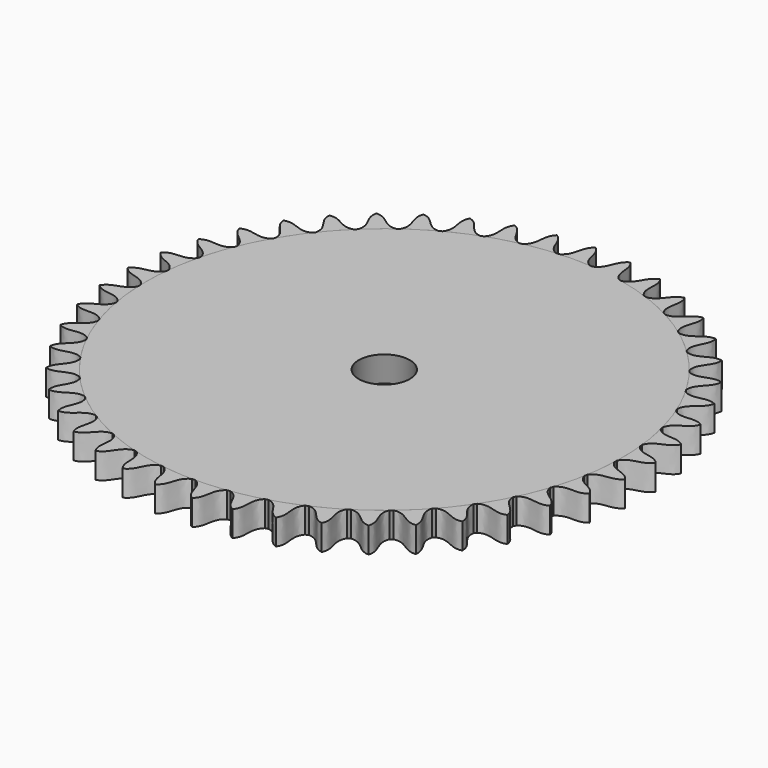
from build123d import *

# Parameters (mm, degrees)
F2_R     = 6
F2_R_2   = 4
F3_DEPTH = 4
F4_COUNT = 45


with BuildPart() as f3:
    # F2 (on Top) → F3 (new body)
    with BuildSketch(Plane.XY):
        with BuildLine():
            ThreePointArc((-2.3528037666, 37.167862426), (-25.4888403137, -27.1533552686), (37.2422566835, 0))
            ThreePointArc((37.2422566835, 0), (27.1533552686, 25.4888403137), (2.3528037666, 37.167862426))
            ThreePointArc((2.3528037666, 37.167862426), (0, 37.2422566835), (-2.3528037666, 37.167862426))
        make_face()
        Circle(F2_R, mode=Mode.SUBTRACT)
        Circle(F2_R)
        Circle(F2_R_2, mode=Mode.SUBTRACT)
        with BuildLine():
            ThreePointArc((-2.3528037666, 37.167862426), (0, 37.2422566835), (2.3528037666, 37.167862426))
            add(Edge.make_bspline(
                [(0, 41.294973545), (1.5, 40.167862426), (0.65, 38.167862426), (2.3528037666, 37.167862426)],
                knots=[0, 0, 0, 0, 4.7506559287, 4.7506559287, 4.7506559287, 4.7506559287], degree=3))
            add(Edge.make_bspline(
                [(0, 41.294973545), (-1.5, 40.167862426), (-0.65, 38.167862426), (-2.3528037666, 37.167862426)],
                knots=[0, 0, 0, 0, 4.7506559287, 4.7506559287, 4.7506559287, 4.7506559287], degree=3))
        make_face()
    extrude(amount=F3_DEPTH)


with BuildPart() as f4_1:
    # F4: instance of F3
    add(f3.part.rotate(Axis((0, 0, 4), (0, 0, 1)), 1 * 360 / F4_COUNT))


with BuildPart() as f4_2:
    # F4: instance of F3
    add(f3.part.rotate(Axis((0, 0, 4), (0, 0, 1)), 2 * 360 / F4_COUNT))


with BuildPart() as f4_3:
    # F4: instance of F3
    add(f3.part.rotate(Axis((0, 0, 4), (0, 0, 1)), 3 * 360 / F4_COUNT))


with BuildPart() as f4_4:
    # F4: instance of F3
    add(f3.part.rotate(Axis((0, 0, 4), (0, 0, 1)), 4 * 360 / F4_COUNT))


with BuildPart() as f4_5:
    # F4: instance of F3
    add(f3.part.rotate(Axis((0, 0, 4), (0, 0, 1)), 5 * 360 / F4_COUNT))


with BuildPart() as f4_6:
    # F4: instance of F3
    add(f3.part.rotate(Axis((0, 0, 4), (0, 0, 1)), 6 * 360 / F4_COUNT))


with BuildPart() as f4_7:
    # F4: instance of F3
    add(f3.part.rotate(Axis((0, 0, 4), (0, 0, 1)), 7 * 360 / F4_COUNT))


with BuildPart() as f4_8:
    # F4: instance of F3
    add(f3.part.rotate(Axis((0, 0, 4), (0, 0, 1)), 8 * 360 / F4_COUNT))


with BuildPart() as f4_9:
    # F4: instance of F3
    add(f3.part.rotate(Axis((0, 0, 4), (0, 0, 1)), 9 * 360 / F4_COUNT))


with BuildPart() as f4_10:
    # F4: instance of F3
    add(f3.part.rotate(Axis((0, 0, 4), (0, 0, 1)), 10 * 360 / F4_COUNT))


with BuildPart() as f4_11:
    # F4: instance of F3
    add(f3.part.rotate(Axis((0, 0, 4), (0, 0, 1)), 11 * 360 / F4_COUNT))


with BuildPart() as f4_12:
    # F4: instance of F3
    add(f3.part.rotate(Axis((0, 0, 4), (0, 0, 1)), 12 * 360 / F4_COUNT))


with BuildPart() as f4_13:
    # F4: instance of F3
    add(f3.part.rotate(Axis((0, 0, 4), (0, 0, 1)), 13 * 360 / F4_COUNT))


with BuildPart() as f4_14:
    # F4: instance of F3
    add(f3.part.rotate(Axis((0, 0, 4), (0, 0, 1)), 14 * 360 / F4_COUNT))


with BuildPart() as f4_15:
    # F4: instance of F3
    add(f3.part.rotate(Axis((0, 0, 4), (0, 0, 1)), 15 * 360 / F4_COUNT))


with BuildPart() as f4_16:
    # F4: instance of F3
    add(f3.part.rotate(Axis((0, 0, 4), (0, 0, 1)), 16 * 360 / F4_COUNT))


with BuildPart() as f4_17:
    # F4: instance of F3
    add(f3.part.rotate(Axis((0, 0, 4), (0, 0, 1)), 17 * 360 / F4_COUNT))


with BuildPart() as f4_18:
    # F4: instance of F3
    add(f3.part.rotate(Axis((0, 0, 4), (0, 0, 1)), 18 * 360 / F4_COUNT))


with BuildPart() as f4_19:
    # F4: instance of F3
    add(f3.part.rotate(Axis((0, 0, 4), (0, 0, 1)), 19 * 360 / F4_COUNT))


with BuildPart() as f4_20:
    # F4: instance of F3
    add(f3.part.rotate(Axis((0, 0, 4), (0, 0, 1)), 20 * 360 / F4_COUNT))


with BuildPart() as f4_21:
    # F4: instance of F3
    add(f3.part.rotate(Axis((0, 0, 4), (0, 0, 1)), 21 * 360 / F4_COUNT))


with BuildPart() as f4_22:
    # F4: instance of F3
    add(f3.part.rotate(Axis((0, 0, 4), (0, 0, 1)), 22 * 360 / F4_COUNT))


with BuildPart() as f4_23:
    # F4: instance of F3
    add(f3.part.rotate(Axis((0, 0, 4), (0, 0, 1)), 23 * 360 / F4_COUNT))


with BuildPart() as f4_24:
    # F4: instance of F3
    add(f3.part.rotate(Axis((0, 0, 4), (0, 0, 1)), 24 * 360 / F4_COUNT))


with BuildPart() as f4_25:
    # F4: instance of F3
    add(f3.part.rotate(Axis((0, 0, 4), (0, 0, 1)), 25 * 360 / F4_COUNT))


with BuildPart() as f4_26:
    # F4: instance of F3
    add(f3.part.rotate(Axis((0, 0, 4), (0, 0, 1)), 26 * 360 / F4_COUNT))


with BuildPart() as f4_27:
    # F4: instance of F3
    add(f3.part.rotate(Axis((0, 0, 4), (0, 0, 1)), 27 * 360 / F4_COUNT))


with BuildPart() as f4_28:
    # F4: instance of F3
    add(f3.part.rotate(Axis((0, 0, 4), (0, 0, 1)), 28 * 360 / F4_COUNT))


with BuildPart() as f4_29:
    # F4: instance of F3
    add(f3.part.rotate(Axis((0, 0, 4), (0, 0, 1)), 29 * 360 / F4_COUNT))


with BuildPart() as f4_30:
    # F4: instance of F3
    add(f3.part.rotate(Axis((0, 0, 4), (0, 0, 1)), 30 * 360 / F4_COUNT))


with BuildPart() as f4_31:
    # F4: instance of F3
    add(f3.part.rotate(Axis((0, 0, 4), (0, 0, 1)), 31 * 360 / F4_COUNT))


with BuildPart() as f4_32:
    # F4: instance of F3
    add(f3.part.rotate(Axis((0, 0, 4), (0, 0, 1)), 32 * 360 / F4_COUNT))


with BuildPart() as f4_33:
    # F4: instance of F3
    add(f3.part.rotate(Axis((0, 0, 4), (0, 0, 1)), 33 * 360 / F4_COUNT))


with BuildPart() as f4_34:
    # F4: instance of F3
    add(f3.part.rotate(Axis((0, 0, 4), (0, 0, 1)), 34 * 360 / F4_COUNT))


with BuildPart() as f4_35:
    # F4: instance of F3
    add(f3.part.rotate(Axis((0, 0, 4), (0, 0, 1)), 35 * 360 / F4_COUNT))


with BuildPart() as f4_36:
    # F4: instance of F3
    add(f3.part.rotate(Axis((0, 0, 4), (0, 0, 1)), 36 * 360 / F4_COUNT))


with BuildPart() as f4_37:
    # F4: instance of F3
    add(f3.part.rotate(Axis((0, 0, 4), (0, 0, 1)), 37 * 360 / F4_COUNT))


with BuildPart() as f4_38:
    # F4: instance of F3
    add(f3.part.rotate(Axis((0, 0, 4), (0, 0, 1)), 38 * 360 / F4_COUNT))


with BuildPart() as f4_39:
    # F4: instance of F3
    add(f3.part.rotate(Axis((0, 0, 4), (0, 0, 1)), 39 * 360 / F4_COUNT))


with BuildPart() as f4_40:
    # F4: instance of F3
    add(f3.part.rotate(Axis((0, 0, 4), (0, 0, 1)), 40 * 360 / F4_COUNT))


with BuildPart() as f4_41:
    # F4: instance of F3
    add(f3.part.rotate(Axis((0, 0, 4), (0, 0, 1)), 41 * 360 / F4_COUNT))


with BuildPart() as f4_42:
    # F4: instance of F3
    add(f3.part.rotate(Axis((0, 0, 4), (0, 0, 1)), 42 * 360 / F4_COUNT))


with BuildPart() as f4_43:
    # F4: instance of F3
    add(f3.part.rotate(Axis((0, 0, 4), (0, 0, 1)), 43 * 360 / F4_COUNT))


with BuildPart() as f4_44:
    # F4: instance of F3
    add(f3.part.rotate(Axis((0, 0, 4), (0, 0, 1)), 44 * 360 / F4_COUNT))


solid = Compound([f3.part, f4_1.part, f4_2.part, f4_3.part, f4_4.part, f4_5.part, f4_6.part, f4_7.part, f4_8.part, f4_9.part, f4_10.part, f4_11.part, f4_12.part, f4_13.part, f4_14.part, f4_15.part, f4_16.part, f4_17.part, f4_18.part, f4_19.part, f4_20.part, f4_21.part, f4_22.part, f4_23.part, f4_24.part, f4_25.part, f4_26.part, f4_27.part, f4_28.part, f4_29.part, f4_30.part, f4_31.part, f4_32.part, f4_33.part, f4_34.part, f4_35.part, f4_36.part, f4_37.part, f4_38.part, f4_39.part, f4_40.part, f4_41.part, f4_42.part, f4_43.part, f4_44.part])
